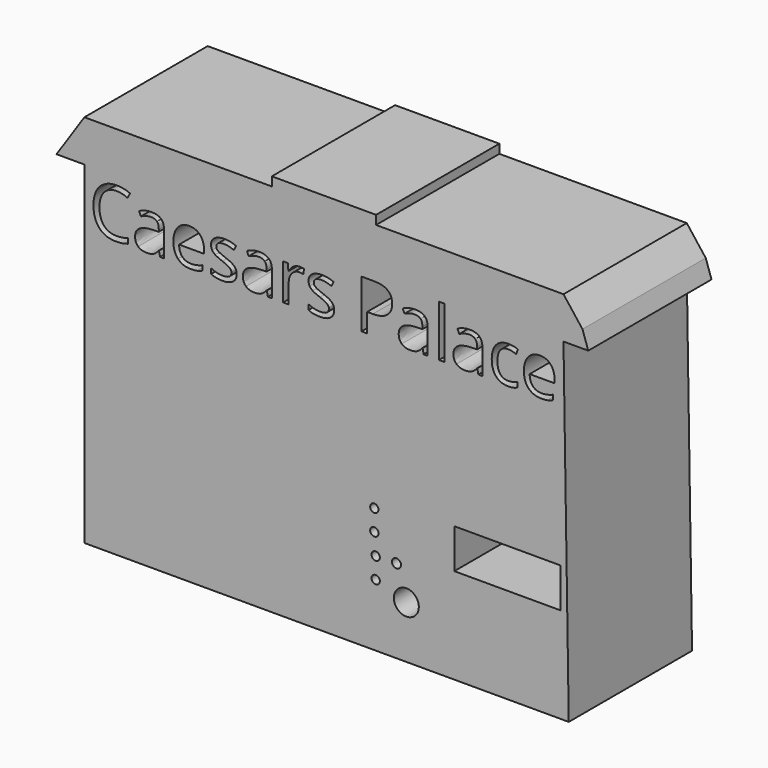
from build123d import *

# Parameters (mm, degrees)
F0_W     = 66.9038857644
F0_H     = 626.8855423356
F1_DEPTH = 1879.6
F2_R     = 54.9444288962
F2_R_2   = 50.8
F3_DEPTH = 4038.6
F4_W     = 1295.4
F4_H     = 482.6
F5_DEPTH = 2717.8
F6_R     = 152.4
F7_DEPTH = 3378.2


# Not quite as in the source:
# - a feature names something its author has since deleted; it is built from what else it names


with BuildPart() as f1:
    # F0 (on Front) → F1 (new body)
    with BuildSketch(Plane.XZ):
        Polygon((208.8753432035, -1016), (549.4310855865, -1016), (6393.364906311, -1016), (6695.2958106995, -1016), (6624.9423027039, -807.6888309717), (6393.364906311, -508), (4107.364906311, -508), (4107.364906311, -399.0220116377), (2835.4310855865, -399.0220116377), (2835.4310855865, -508), (549.4310855865, -508), align=None)
        Polygon((549.4310855865, -1016), (549.4310855865, -5080), (6457.6897621155, -5080), (6393.364906311, -1016), align=None)
        with BuildLine():
            add(Edge.make_bspline(
                [(1076.286761918, -1203.7427777217), (1009.3828761536, -1172.4178369881), (942.4789903892, -1172.4178369881)],
                knots=[0, 0, 0, 1, 1, 1], degree=2))
            add(Edge.make_bspline(
                [(942.4789903892, -1172.4178369881), (845.4103468814, -1172.4178369881), (789.2059264705, -1237.0658113828)],
                knots=[0, 0, 0, 1, 1, 1], degree=2))
            add(Edge.make_bspline(
                [(789.2059264705, -1237.0658113828), (733.0015060595, -1301.7137857775), (733.0015060595, -1414.1226265993)],
                knots=[0, 0, 0, 1, 1, 1], degree=2))
            add(Edge.make_bspline(
                [(733.0015060595, -1414.1226265993), (733.0015060595, -1529.6252887282), (787.207833543, -1592.7263524694)],
                knots=[0, 0, 0, 1, 1, 1], degree=2))
            add(Edge.make_bspline(
                [(787.207833543, -1592.7263524694), (841.4141610265, -1655.8274162105), (941.7055350625, -1655.8274162105)],
                knots=[0, 0, 0, 1, 1, 1], degree=2))
            add(Edge.make_bspline(
                [(941.7055350625, -1655.8274162105), (1003.3241427607, -1655.8274162105), (1082.3454953109, -1633.6550301769)],
                knots=[0, 0, 0, 1, 1, 1], degree=2))
            Line((1082.3454953109, -1633.6550301769), (1082.3454953109, -1693.5978180004))
            add(Edge.make_bspline(
                [(1082.3454953109, -1693.5978180004), (1021.1136152761, -1716.672568582), (931.2638881513, -1716.672568582)],
                knots=[0, 0, 0, 1, 1, 1], degree=2))
            add(Edge.make_bspline(
                [(931.2638881513, -1716.672568582), (801.1944840352, -1716.672568582), (730.4877762476, -1637.6512160318)],
                knots=[0, 0, 0, 1, 1, 1], degree=2))
            add(Edge.make_bspline(
                [(730.4877762476, -1637.6512160318), (659.78106846, -1558.6298634816), (659.78106846, -1413.2202620515)],
                knots=[0, 0, 0, 1, 1, 1], degree=2))
            add(Edge.make_bspline(
                [(659.78106846, -1413.2202620515), (659.78106846, -1322.2103519365), (693.8131028372, -1253.7595555186)],
                knots=[0, 0, 0, 1, 1, 1], degree=2))
            add(Edge.make_bspline(
                [(693.8131028372, -1253.7595555186), (727.8451372145, -1185.3087591007), (792.1063839458, -1148.247358027)],
                knots=[0, 0, 0, 1, 1, 1], degree=2))
            add(Edge.make_bspline(
                [(792.1063839458, -1148.247358027), (856.3676306771, -1111.1859569533), (943.3813549371, -1111.1859569533)],
                knots=[0, 0, 0, 1, 1, 1], degree=2))
            add(Edge.make_bspline(
                [(943.3813549371, -1111.1859569533), (1035.9381757056, -1111.1859569533), (1105.2913366713, -1144.9601728883)],
                knots=[0, 0, 0, 1, 1, 1], degree=2))
            Line((1105.2913366713, -1144.9601728883), (1076.286761918, -1203.7427777217))
        make_face(mode=Mode.SUBTRACT)
        with BuildLine():
            Line((1521.9259393505, -1708.5512876511), (1472.295889217, -1708.5512876511))
            Line((1472.295889217, -1708.5512876511), (1459.018239441, -1645.6435877416))
            Line((1459.018239441, -1645.6435877416), (1455.7955089129, -1645.6435877416))
            add(Edge.make_bspline(
                [(1455.7955089129, -1645.6435877416), (1422.7947483046, -1687.1523569442), (1389.9873515281, -1701.9124627631)],
                knots=[0, 0, 0, 1, 1, 1], degree=2))
            add(Edge.make_bspline(
                [(1389.9873515281, -1701.9124627631), (1357.1799547515, -1716.672568582), (1307.9366322814, -1716.672568582)],
                knots=[0, 0, 0, 1, 1, 1], degree=2))
            add(Edge.make_bspline(
                [(1307.9366322814, -1716.672568582), (1242.3218387283, -1716.672568582), (1205.0670738228, -1682.7694434259)],
                knots=[0, 0, 0, 1, 1, 1], degree=2))
            add(Edge.make_bspline(
                [(1205.0670738228, -1682.7694434259), (1167.8123089174, -1648.8663182697), (1167.8123089174, -1586.4742552448)],
                knots=[0, 0, 0, 1, 1, 1], degree=2))
            add(Edge.make_bspline(
                [(1167.8123089174, -1586.4742552448), (1167.8123089174, -1452.7953929371), (1381.6727067654, -1446.3499318808)],
                knots=[0, 0, 0, 1, 1, 1], degree=2))
            Line((1381.6727067654, -1446.3499318808), (1456.5689642396, -1443.9006566794))
            Line((1456.5689642396, -1443.9006566794), (1456.5689642396, -1416.4429925796))
            add(Edge.make_bspline(
                [(1456.5689642396, -1416.4429925796), (1456.5689642396, -1364.4925764658), (1434.2676689848, -1339.7420060097)],
                knots=[0, 0, 0, 1, 1, 1], degree=2))
            add(Edge.make_bspline(
                [(1434.2676689848, -1339.7420060097), (1411.96637373, -1314.9914355535), (1362.7230512599, -1314.9914355535)],
                knots=[0, 0, 0, 1, 1, 1], degree=2))
            add(Edge.make_bspline(
                [(1362.7230512599, -1314.9914355535), (1307.549904618, -1314.9914355535), (1237.93892521, -1348.7656514885)],
                knots=[0, 0, 0, 1, 1, 1], degree=2))
            Line((1237.93892521, -1348.7656514885), (1217.3134498298, -1297.5886907015))
            add(Edge.make_bspline(
                [(1217.3134498298, -1297.5886907015), (1249.9274827747, -1279.9281274072), (1288.7936129442, -1269.8732081594)],
                knots=[0, 0, 0, 1, 1, 1], degree=2))
            add(Edge.make_bspline(
                [(1288.7936129442, -1269.8732081594), (1327.6597431137, -1259.8182889115), (1366.8481463359, -1259.8182889115)],
                knots=[0, 0, 0, 1, 1, 1], degree=2))
            add(Edge.make_bspline(
                [(1366.8481463359, -1259.8182889115), (1445.740589665, -1259.8182889115), (1483.8332645078, -1294.8171424472)],
                knots=[0, 0, 0, 1, 1, 1], degree=2))
            add(Edge.make_bspline(
                [(1483.8332645078, -1294.8171424472), (1521.9259393505, -1329.815995983), (1521.9259393505, -1407.1615286585)],
                knots=[0, 0, 0, 1, 1, 1], degree=2))
            Line((1521.9259393505, -1407.1615286585), (1521.9259393505, -1708.5512876511))
        make_face(mode=Mode.SUBTRACT)
        with BuildLine():
            add(Edge.make_bspline(
                [(1922.4468893889, -1709.9692890834), (1890.864130213, -1716.672568582), (1846.1326304823, -1716.672568582)],
                knots=[0, 0, 0, 1, 1, 1], degree=2))
            add(Edge.make_bspline(
                [(1846.1326304823, -1716.672568582), (1748.2905316477, -1716.672568582), (1691.6349289628, -1656.9875992007)],
                knots=[0, 0, 0, 1, 1, 1], degree=2))
            add(Edge.make_bspline(
                [(1691.6349289628, -1656.9875992007), (1634.979326278, -1597.3026298193), (1634.979326278, -1491.4681592749)],
                knots=[0, 0, 0, 1, 1, 1], degree=2))
            add(Edge.make_bspline(
                [(1634.979326278, -1491.4681592749), (1634.979326278, -1384.6024149615), (1687.5742884974, -1321.7591696626)],
                knots=[0, 0, 0, 1, 1, 1], degree=2))
            add(Edge.make_bspline(
                [(1687.5742884974, -1321.7591696626), (1740.1692507168, -1258.9159243637), (1828.8587948514, -1258.9159243637)],
                knots=[0, 0, 0, 1, 1, 1], degree=2))
            add(Edge.make_bspline(
                [(1828.8587948514, -1258.9159243637), (1911.7474240354, -1258.9159243637), (1960.0883819577, -1313.5089795105)],
                knots=[0, 0, 0, 1, 1, 1], degree=2))
            add(Edge.make_bspline(
                [(1960.0883819577, -1313.5089795105), (2008.4293398799, -1368.1020346574), (2008.4293398799, -1457.5650341188)],
                knots=[0, 0, 0, 1, 1, 1], degree=2))
            Line((2008.4293398799, -1457.5650341188), (2008.4293398799, -1499.8472586481))
            Line((2008.4293398799, -1499.8472586481), (1704.3324872437, -1499.8472586481))
            add(Edge.make_bspline(
                [(1704.3324872437, -1499.8472586481), (1706.3950347818, -1577.5795189871), (1743.6497996872, -1617.8636505889)],
                knots=[0, 0, 0, 1, 1, 1], degree=2))
            add(Edge.make_bspline(
                [(1743.6497996872, -1617.8636505889), (1780.9045645926, -1658.1477821908), (1848.5819056837, -1658.1477821908)],
                knots=[0, 0, 0, 1, 1, 1], degree=2))
            add(Edge.make_bspline(
                [(1848.5819056837, -1658.1477821908), (1919.8687049664, -1658.1477821908), (1989.4796843744, -1628.3697521107)],
                knots=[0, 0, 0, 1, 1, 1], degree=2))
            Line((1989.4796843744, -1628.3697521107), (1989.4796843744, -1688.054721492))
            add(Edge.make_bspline(
                [(1989.4796843744, -1688.054721492), (1954.0296485648, -1703.2660095849), (1922.4468893889, -1709.9692890834)],
                knots=[0, 0, 0, 1, 1, 1], degree=2))
        make_face(mode=Mode.SUBTRACT)
        with BuildLine():
            add(Edge.make_bspline(
                [(2379.6878967227, -1515.1874559621), (2407.2744700437, -1544.1920307154), (2407.2744700437, -1588.1500751194)],
                knots=[0, 0, 0, 1, 1, 1], degree=2))
            add(Edge.make_bspline(
                [(2407.2744700437, -1588.1500751194), (2407.2744700437, -1649.7686828176), (2361.3827873228, -1683.2206256998)],
                knots=[0, 0, 0, 1, 1, 1], degree=2))
            add(Edge.make_bspline(
                [(2361.3827873228, -1683.2206256998), (2315.491104602, -1716.672568582), (2232.4735661969, -1716.672568582)],
                knots=[0, 0, 0, 1, 1, 1], degree=2))
            add(Edge.make_bspline(
                [(2232.4735661969, -1716.672568582), (2144.6863866101, -1716.672568582), (2095.5719733611, -1688.8281768188)],
                knots=[0, 0, 0, 1, 1, 1], degree=2))
            Line((2095.5719733611, -1688.8281768188), (2095.5719733611, -1626.8228414572))
            add(Edge.make_bspline(
                [(2095.5719733611, -1626.8228414572), (2127.4125509792, -1642.9364940979), (2163.8294059473, -1652.1535034084)],
                knots=[0, 0, 0, 1, 1, 1], degree=2))
            add(Edge.make_bspline(
                [(2163.8294059473, -1652.1535034084), (2200.2462609154, -1661.370512719), (2234.1493860715, -1661.370512719)],
                knots=[0, 0, 0, 1, 1, 1], degree=2))
            add(Edge.make_bspline(
                [(2234.1493860715, -1661.370512719), (2286.4865298486, -1661.370512719), (2314.6531946647, -1644.6767685831)],
                knots=[0, 0, 0, 1, 1, 1], degree=2))
            add(Edge.make_bspline(
                [(2314.6531946647, -1644.6767685831), (2342.8198594807, -1627.9830244473), (2342.8198594807, -1593.6931716278)],
                knots=[0, 0, 0, 1, 1, 1], degree=2))
            add(Edge.make_bspline(
                [(2342.8198594807, -1593.6931716278), (2342.8198594807, -1567.9113274026), (2320.5185642259, -1549.6062180027)],
                knots=[0, 0, 0, 1, 1, 1], degree=2))
            add(Edge.make_bspline(
                [(2320.5185642259, -1549.6062180027), (2298.2172689711, -1531.3011086028), (2233.2470215236, -1506.2927197044)],
                knots=[0, 0, 0, 1, 1, 1], degree=2))
            add(Edge.make_bspline(
                [(2233.2470215236, -1506.2927197044), (2171.6284138254, -1483.346878344), (2145.6532057685, -1466.2019519342)],
                knots=[0, 0, 0, 1, 1, 1], degree=2))
            add(Edge.make_bspline(
                [(2145.6532057685, -1466.2019519342), (2119.6779977116, -1449.0570255245), (2106.9804394307, -1427.3358217648)],
                knots=[0, 0, 0, 1, 1, 1], degree=2))
            add(Edge.make_bspline(
                [(2106.9804394307, -1427.3358217648), (2094.2828811498, -1405.614618005), (2094.2828811498, -1375.4498602615)],
                knots=[0, 0, 0, 1, 1, 1], degree=2))
            add(Edge.make_bspline(
                [(2094.2828811498, -1375.4498602615), (2094.2828811498, -1321.4368966098), (2138.2409255538, -1290.1764104867)],
                knots=[0, 0, 0, 1, 1, 1], degree=2))
            add(Edge.make_bspline(
                [(2138.2409255538, -1290.1764104867), (2182.1989699577, -1258.9159243637), (2258.6421380854, -1258.9159243637)],
                knots=[0, 0, 0, 1, 1, 1], degree=2))
            add(Edge.make_bspline(
                [(2258.6421380854, -1258.9159243637), (2329.9289373681, -1258.9159243637), (2398.1219153437, -1287.920499117)],
                knots=[0, 0, 0, 1, 1, 1], degree=2))
            Line((2398.1219153437, -1287.920499117), (2374.2737094354, -1342.3201904322))
            add(Edge.make_bspline(
                [(2374.2737094354, -1342.3201904322), (2307.8854605556, -1314.9914355535), (2253.8724969038, -1314.9914355535)],
                knots=[0, 0, 0, 1, 1, 1], degree=2))
            add(Edge.make_bspline(
                [(2253.8724969038, -1314.9914355535), (2206.3049943083, -1314.9914355535), (2182.1345153472, -1329.8804505935)],
                knots=[0, 0, 0, 1, 1, 1], degree=2))
            add(Edge.make_bspline(
                [(2182.1345153472, -1329.8804505935), (2157.964036386, -1344.7694656336), (2157.964036386, -1370.9380375221)],
                knots=[0, 0, 0, 1, 1, 1], degree=2))
            add(Edge.make_bspline(
                [(2157.964036386, -1370.9380375221), (2157.964036386, -1388.7275100375), (2167.0521364754, -1401.1672498762)],
                knots=[0, 0, 0, 1, 1, 1], degree=2))
            add(Edge.make_bspline(
                [(2167.0521364754, -1401.1672498762), (2176.1402365648, -1413.6069897148), (2196.2500750605, -1424.8865465634)],
                knots=[0, 0, 0, 1, 1, 1], degree=2))
            add(Edge.make_bspline(
                [(2196.2500750605, -1424.8865465634), (2216.3599135561, -1436.1661034119), (2273.595607736, -1457.5650341188)],
                knots=[0, 0, 0, 1, 1, 1], degree=2))
            add(Edge.make_bspline(
                [(2273.595607736, -1457.5650341188), (2352.1013234018, -1486.1828812088), (2379.6878967227, -1515.1874559621)],
                knots=[0, 0, 0, 1, 1, 1], degree=2))
        make_face(mode=Mode.SUBTRACT)
        with BuildLine():
            Line((2837.1867224988, -1708.5512876511), (2787.5566723653, -1708.5512876511))
            Line((2787.5566723653, -1708.5512876511), (2774.2790225893, -1645.6435877416))
            Line((2774.2790225893, -1645.6435877416), (2771.0562920612, -1645.6435877416))
            add(Edge.make_bspline(
                [(2771.0562920612, -1645.6435877416), (2738.0555314529, -1687.1523569442), (2705.2481346764, -1701.9124627631)],
                knots=[0, 0, 0, 1, 1, 1], degree=2))
            add(Edge.make_bspline(
                [(2705.2481346764, -1701.9124627631), (2672.4407378998, -1716.672568582), (2623.1974154297, -1716.672568582)],
                knots=[0, 0, 0, 1, 1, 1], degree=2))
            add(Edge.make_bspline(
                [(2623.1974154297, -1716.672568582), (2557.5826218766, -1716.672568582), (2520.3278569712, -1682.7694434259)],
                knots=[0, 0, 0, 1, 1, 1], degree=2))
            add(Edge.make_bspline(
                [(2520.3278569712, -1682.7694434259), (2483.0730920658, -1648.8663182697), (2483.0730920658, -1586.4742552448)],
                knots=[0, 0, 0, 1, 1, 1], degree=2))
            add(Edge.make_bspline(
                [(2483.0730920658, -1586.4742552448), (2483.0730920658, -1452.7953929371), (2696.9334899137, -1446.3499318808)],
                knots=[0, 0, 0, 1, 1, 1], degree=2))
            Line((2696.9334899137, -1446.3499318808), (2771.8297473879, -1443.9006566794))
            Line((2771.8297473879, -1443.9006566794), (2771.8297473879, -1416.4429925796))
            add(Edge.make_bspline(
                [(2771.8297473879, -1416.4429925796), (2771.8297473879, -1364.4925764658), (2749.5284521331, -1339.7420060097)],
                knots=[0, 0, 0, 1, 1, 1], degree=2))
            add(Edge.make_bspline(
                [(2749.5284521331, -1339.7420060097), (2727.2271568783, -1314.9914355535), (2677.9838344082, -1314.9914355535)],
                knots=[0, 0, 0, 1, 1, 1], degree=2))
            add(Edge.make_bspline(
                [(2677.9838344082, -1314.9914355535), (2622.8106877663, -1314.9914355535), (2553.1997083583, -1348.7656514885)],
                knots=[0, 0, 0, 1, 1, 1], degree=2))
            Line((2553.1997083583, -1348.7656514885), (2532.5742329781, -1297.5886907015))
            add(Edge.make_bspline(
                [(2532.5742329781, -1297.5886907015), (2565.188265923, -1279.9281274072), (2604.0543960925, -1269.8732081594)],
                knots=[0, 0, 0, 1, 1, 1], degree=2))
            add(Edge.make_bspline(
                [(2604.0543960925, -1269.8732081594), (2642.920526262, -1259.8182889115), (2682.1089294843, -1259.8182889115)],
                knots=[0, 0, 0, 1, 1, 1], degree=2))
            add(Edge.make_bspline(
                [(2682.1089294843, -1259.8182889115), (2761.0013728134, -1259.8182889115), (2799.0940476561, -1294.8171424472)],
                knots=[0, 0, 0, 1, 1, 1], degree=2))
            add(Edge.make_bspline(
                [(2799.0940476561, -1294.8171424472), (2837.1867224988, -1329.815995983), (2837.1867224988, -1407.1615286585)],
                knots=[0, 0, 0, 1, 1, 1], degree=2))
            Line((2837.1867224988, -1407.1615286585), (2837.1867224988, -1708.5512876511))
        make_face(mode=Mode.SUBTRACT)
        with BuildLine():
            add(Edge.make_bspline(
                [(3100.1615335958, -1282.312947998), (3134.8381140787, -1258.9159243637), (3176.3468832812, -1258.9159243637)],
                knots=[0, 0, 0, 1, 1, 1], degree=2))
            add(Edge.make_bspline(
                [(3176.3468832812, -1258.9159243637), (3205.738185698, -1258.9159243637), (3229.0707547218, -1263.8144747665)],
                knots=[0, 0, 0, 1, 1, 1], degree=2))
            Line((3229.0707547218, -1263.8144747665), (3219.7892908007, -1325.819810128))
            add(Edge.make_bspline(
                [(3219.7892908007, -1325.819810128), (3192.460535922, -1319.7610767351), (3171.4483328785, -1319.7610767351)],
                knots=[0, 0, 0, 1, 1, 1], degree=2))
            add(Edge.make_bspline(
                [(3171.4483328785, -1319.7610767351), (3117.82209689, -1319.7610767351), (3079.7938766579, -1363.2679388651)],
                knots=[0, 0, 0, 1, 1, 1], degree=2))
            add(Edge.make_bspline(
                [(3079.7938766579, -1363.2679388651), (3041.7656564257, -1406.7748009952), (3041.7656564257, -1471.6161392215)],
                knots=[0, 0, 0, 1, 1, 1], degree=2))
            Line((3041.7656564257, -1471.6161392215), (3041.7656564257, -1708.5512876511))
            Line((3041.7656564257, -1708.5512876511), (2974.8617706613, -1708.5512876511))
            Line((2974.8617706613, -1708.5512876511), (2974.8617706613, -1267.0372052946))
            Line((2974.8617706613, -1267.0372052946), (3030.0349173033, -1267.0372052946))
            Line((3030.0349173033, -1267.0372052946), (3037.7694705708, -1348.7656514885))
            Line((3037.7694705708, -1348.7656514885), (3040.992201099, -1348.7656514885))
            add(Edge.make_bspline(
                [(3040.992201099, -1348.7656514885), (3065.4849531129, -1305.7099716324), (3100.1615335958, -1282.312947998)],
                knots=[0, 0, 0, 1, 1, 1], degree=2))
        make_face(mode=Mode.SUBTRACT)
        with BuildLine():
            add(Edge.make_bspline(
                [(3568.8754616098, -1515.1874559621), (3596.4620349308, -1544.1920307154), (3596.4620349308, -1588.1500751194)],
                knots=[0, 0, 0, 1, 1, 1], degree=2))
            add(Edge.make_bspline(
                [(3596.4620349308, -1588.1500751194), (3596.4620349308, -1649.7686828176), (3550.5703522099, -1683.2206256998)],
                knots=[0, 0, 0, 1, 1, 1], degree=2))
            add(Edge.make_bspline(
                [(3550.5703522099, -1683.2206256998), (3504.6786694891, -1716.672568582), (3421.661131084, -1716.672568582)],
                knots=[0, 0, 0, 1, 1, 1], degree=2))
            add(Edge.make_bspline(
                [(3421.661131084, -1716.672568582), (3333.8739514972, -1716.672568582), (3284.7595382482, -1688.8281768188)],
                knots=[0, 0, 0, 1, 1, 1], degree=2))
            Line((3284.7595382482, -1688.8281768188), (3284.7595382482, -1626.8228414572))
            add(Edge.make_bspline(
                [(3284.7595382482, -1626.8228414572), (3316.6001158663, -1642.9364940979), (3353.0169708344, -1652.1535034084)],
                knots=[0, 0, 0, 1, 1, 1], degree=2))
            add(Edge.make_bspline(
                [(3353.0169708344, -1652.1535034084), (3389.4338258025, -1661.370512719), (3423.3369509586, -1661.370512719)],
                knots=[0, 0, 0, 1, 1, 1], degree=2))
            add(Edge.make_bspline(
                [(3423.3369509586, -1661.370512719), (3475.6740947358, -1661.370512719), (3503.8407595518, -1644.6767685831)],
                knots=[0, 0, 0, 1, 1, 1], degree=2))
            add(Edge.make_bspline(
                [(3503.8407595518, -1644.6767685831), (3532.0074243678, -1627.9830244473), (3532.0074243678, -1593.6931716278)],
                knots=[0, 0, 0, 1, 1, 1], degree=2))
            add(Edge.make_bspline(
                [(3532.0074243678, -1593.6931716278), (3532.0074243678, -1567.9113274026), (3509.706129113, -1549.6062180027)],
                knots=[0, 0, 0, 1, 1, 1], degree=2))
            add(Edge.make_bspline(
                [(3509.706129113, -1549.6062180027), (3487.4048338582, -1531.3011086028), (3422.4345864107, -1506.2927197044)],
                knots=[0, 0, 0, 1, 1, 1], degree=2))
            add(Edge.make_bspline(
                [(3422.4345864107, -1506.2927197044), (3360.8159787125, -1483.346878344), (3334.8407706556, -1466.2019519342)],
                knots=[0, 0, 0, 1, 1, 1], degree=2))
            add(Edge.make_bspline(
                [(3334.8407706556, -1466.2019519342), (3308.8655625987, -1449.0570255245), (3296.1680043178, -1427.3358217648)],
                knots=[0, 0, 0, 1, 1, 1], degree=2))
            add(Edge.make_bspline(
                [(3296.1680043178, -1427.3358217648), (3283.4704460369, -1405.614618005), (3283.4704460369, -1375.4498602615)],
                knots=[0, 0, 0, 1, 1, 1], degree=2))
            add(Edge.make_bspline(
                [(3283.4704460369, -1375.4498602615), (3283.4704460369, -1321.4368966098), (3327.4284904409, -1290.1764104867)],
                knots=[0, 0, 0, 1, 1, 1], degree=2))
            add(Edge.make_bspline(
                [(3327.4284904409, -1290.1764104867), (3371.3865348448, -1258.9159243637), (3447.8297029725, -1258.9159243637)],
                knots=[0, 0, 0, 1, 1, 1], degree=2))
            add(Edge.make_bspline(
                [(3447.8297029725, -1258.9159243637), (3519.1165022552, -1258.9159243637), (3587.3094802308, -1287.920499117)],
                knots=[0, 0, 0, 1, 1, 1], degree=2))
            Line((3587.3094802308, -1287.920499117), (3563.4612743225, -1342.3201904322))
            add(Edge.make_bspline(
                [(3563.4612743225, -1342.3201904322), (3497.0730254427, -1314.9914355535), (3443.0600617909, -1314.9914355535)],
                knots=[0, 0, 0, 1, 1, 1], degree=2))
            add(Edge.make_bspline(
                [(3443.0600617909, -1314.9914355535), (3395.4925591954, -1314.9914355535), (3371.3220802343, -1329.8804505935)],
                knots=[0, 0, 0, 1, 1, 1], degree=2))
            add(Edge.make_bspline(
                [(3371.3220802343, -1329.8804505935), (3347.1516012732, -1344.7694656336), (3347.1516012732, -1370.9380375221)],
                knots=[0, 0, 0, 1, 1, 1], degree=2))
            add(Edge.make_bspline(
                [(3347.1516012732, -1370.9380375221), (3347.1516012732, -1388.7275100375), (3356.2397013625, -1401.1672498762)],
                knots=[0, 0, 0, 1, 1, 1], degree=2))
            add(Edge.make_bspline(
                [(3356.2397013625, -1401.1672498762), (3365.3278014519, -1413.6069897148), (3385.4376399476, -1424.8865465634)],
                knots=[0, 0, 0, 1, 1, 1], degree=2))
            add(Edge.make_bspline(
                [(3385.4376399476, -1424.8865465634), (3405.5474784432, -1436.1661034119), (3462.7831726232, -1457.5650341188)],
                knots=[0, 0, 0, 1, 1, 1], degree=2))
            add(Edge.make_bspline(
                [(3462.7831726232, -1457.5650341188), (3541.2888882889, -1486.1828812088), (3568.8754616098, -1515.1874559621)],
                knots=[0, 0, 0, 1, 1, 1], degree=2))
        make_face(mode=Mode.SUBTRACT)
        with BuildLine():
            add(Edge.make_bspline(
                [(4082.4497985757, -1119.5650563265), (4303.1423851434, -1119.5650563265), (4303.1423851434, -1291.1432296452)],
                knots=[0, 0, 0, 1, 1, 1], degree=2))
            add(Edge.make_bspline(
                [(4303.1423851434, -1291.1432296452), (4303.1423851434, -1380.6062291066), (4242.1038689402, -1428.7538231971)],
                knots=[0, 0, 0, 1, 1, 1], degree=2))
            add(Edge.make_bspline(
                [(4242.1038689402, -1428.7538231971), (4181.0653527371, -1476.9014172877), (4067.4963289251, -1476.9014172877)],
                knots=[0, 0, 0, 1, 1, 1], degree=2))
            Line((4067.4963289251, -1476.9014172877), (3998.1431679593, -1476.9014172877))
            Line((3998.1431679593, -1476.9014172877), (3998.1431679593, -1708.5512876511))
            Line((3998.1431679593, -1708.5512876511), (3929.6923715414, -1708.5512876511))
            Line((3929.6923715414, -1708.5512876511), (3929.6923715414, -1119.5650563265))
            Line((3929.6923715414, -1119.5650563265), (4082.4497985757, -1119.5650563265))
        make_face(mode=Mode.SUBTRACT)
        with BuildLine():
            Line((4737.4375511168, -1708.5512876511), (4687.8075009833, -1708.5512876511))
            Line((4687.8075009833, -1708.5512876511), (4674.5298512073, -1645.6435877416))
            Line((4674.5298512073, -1645.6435877416), (4671.3071206792, -1645.6435877416))
            add(Edge.make_bspline(
                [(4671.3071206792, -1645.6435877416), (4638.3063600709, -1687.1523569442), (4605.4989632943, -1701.9124627631)],
                knots=[0, 0, 0, 1, 1, 1], degree=2))
            add(Edge.make_bspline(
                [(4605.4989632943, -1701.9124627631), (4572.6915665178, -1716.672568582), (4523.4482440477, -1716.672568582)],
                knots=[0, 0, 0, 1, 1, 1], degree=2))
            add(Edge.make_bspline(
                [(4523.4482440477, -1716.672568582), (4457.8334504945, -1716.672568582), (4420.5786855891, -1682.7694434259)],
                knots=[0, 0, 0, 1, 1, 1], degree=2))
            add(Edge.make_bspline(
                [(4420.5786855891, -1682.7694434259), (4383.3239206837, -1648.8663182697), (4383.3239206837, -1586.4742552448)],
                knots=[0, 0, 0, 1, 1, 1], degree=2))
            add(Edge.make_bspline(
                [(4383.3239206837, -1586.4742552448), (4383.3239206837, -1452.7953929371), (4597.1843185317, -1446.3499318808)],
                knots=[0, 0, 0, 1, 1, 1], degree=2))
            Line((4597.1843185317, -1446.3499318808), (4672.0805760059, -1443.9006566794))
            Line((4672.0805760059, -1443.9006566794), (4672.0805760059, -1416.4429925796))
            add(Edge.make_bspline(
                [(4672.0805760059, -1416.4429925796), (4672.0805760059, -1364.4925764658), (4649.7792807511, -1339.7420060097)],
                knots=[0, 0, 0, 1, 1, 1], degree=2))
            add(Edge.make_bspline(
                [(4649.7792807511, -1339.7420060097), (4627.4779854963, -1314.9914355535), (4578.2346630262, -1314.9914355535)],
                knots=[0, 0, 0, 1, 1, 1], degree=2))
            add(Edge.make_bspline(
                [(4578.2346630262, -1314.9914355535), (4523.0615163843, -1314.9914355535), (4453.4505369763, -1348.7656514885)],
                knots=[0, 0, 0, 1, 1, 1], degree=2))
            Line((4453.4505369763, -1348.7656514885), (4432.8250615961, -1297.5886907015))
            add(Edge.make_bspline(
                [(4432.8250615961, -1297.5886907015), (4465.439094541, -1279.9281274072), (4504.3052247105, -1269.8732081594)],
                knots=[0, 0, 0, 1, 1, 1], degree=2))
            add(Edge.make_bspline(
                [(4504.3052247105, -1269.8732081594), (4543.1713548799, -1259.8182889115), (4582.3597581022, -1259.8182889115)],
                knots=[0, 0, 0, 1, 1, 1], degree=2))
            add(Edge.make_bspline(
                [(4582.3597581022, -1259.8182889115), (4661.2522014313, -1259.8182889115), (4699.3448762741, -1294.8171424472)],
                knots=[0, 0, 0, 1, 1, 1], degree=2))
            add(Edge.make_bspline(
                [(4699.3448762741, -1294.8171424472), (4737.4375511168, -1329.815995983), (4737.4375511168, -1407.1615286585)],
                knots=[0, 0, 0, 1, 1, 1], degree=2))
            Line((4737.4375511168, -1407.1615286585), (4737.4375511168, -1708.5512876511))
        make_face(mode=Mode.SUBTRACT)
        with Locations((4908.5645421615, -1395.1085164833)):
            Rectangle(F0_W, F0_H, mode=Mode.SUBTRACT)
        with BuildLine():
            Line((5404.9294981071, -1708.5512876511), (5355.2994479736, -1708.5512876511))
            Line((5355.2994479736, -1708.5512876511), (5342.0217981976, -1645.6435877416))
            Line((5342.0217981976, -1645.6435877416), (5338.7990676694, -1645.6435877416))
            add(Edge.make_bspline(
                [(5338.7990676694, -1645.6435877416), (5305.7983070612, -1687.1523569442), (5272.9909102846, -1701.9124627631)],
                knots=[0, 0, 0, 1, 1, 1], degree=2))
            add(Edge.make_bspline(
                [(5272.9909102846, -1701.9124627631), (5240.1835135081, -1716.672568582), (5190.940191038, -1716.672568582)],
                knots=[0, 0, 0, 1, 1, 1], degree=2))
            add(Edge.make_bspline(
                [(5190.940191038, -1716.672568582), (5125.3253974848, -1716.672568582), (5088.0706325794, -1682.7694434259)],
                knots=[0, 0, 0, 1, 1, 1], degree=2))
            add(Edge.make_bspline(
                [(5088.0706325794, -1682.7694434259), (5050.815867674, -1648.8663182697), (5050.815867674, -1586.4742552448)],
                knots=[0, 0, 0, 1, 1, 1], degree=2))
            add(Edge.make_bspline(
                [(5050.815867674, -1586.4742552448), (5050.815867674, -1452.7953929371), (5264.676265522, -1446.3499318808)],
                knots=[0, 0, 0, 1, 1, 1], degree=2))
            Line((5264.676265522, -1446.3499318808), (5339.5725229962, -1443.9006566794))
            Line((5339.5725229962, -1443.9006566794), (5339.5725229962, -1416.4429925796))
            add(Edge.make_bspline(
                [(5339.5725229962, -1416.4429925796), (5339.5725229962, -1364.4925764658), (5317.2712277414, -1339.7420060097)],
                knots=[0, 0, 0, 1, 1, 1], degree=2))
            add(Edge.make_bspline(
                [(5317.2712277414, -1339.7420060097), (5294.9699324866, -1314.9914355535), (5245.7266100165, -1314.9914355535)],
                knots=[0, 0, 0, 1, 1, 1], degree=2))
            add(Edge.make_bspline(
                [(5245.7266100165, -1314.9914355535), (5190.5534633746, -1314.9914355535), (5120.9424839666, -1348.7656514885)],
                knots=[0, 0, 0, 1, 1, 1], degree=2))
            Line((5120.9424839666, -1348.7656514885), (5100.3170085864, -1297.5886907015))
            add(Edge.make_bspline(
                [(5100.3170085864, -1297.5886907015), (5132.9310415313, -1279.9281274072), (5171.7971717007, -1269.8732081594)],
                knots=[0, 0, 0, 1, 1, 1], degree=2))
            add(Edge.make_bspline(
                [(5171.7971717007, -1269.8732081594), (5210.6633018702, -1259.8182889115), (5249.8517050925, -1259.8182889115)],
                knots=[0, 0, 0, 1, 1, 1], degree=2))
            add(Edge.make_bspline(
                [(5249.8517050925, -1259.8182889115), (5328.7441484216, -1259.8182889115), (5366.8368232643, -1294.8171424472)],
                knots=[0, 0, 0, 1, 1, 1], degree=2))
            add(Edge.make_bspline(
                [(5366.8368232643, -1294.8171424472), (5404.9294981071, -1329.815995983), (5404.9294981071, -1407.1615286585)],
                knots=[0, 0, 0, 1, 1, 1], degree=2))
            Line((5404.9294981071, -1407.1615286585), (5404.9294981071, -1708.5512876511))
        make_face(mode=Mode.SUBTRACT)
        with BuildLine():
            add(Edge.make_bspline(
                [(5830.587746265, -1693.5978180004), (5786.3718834188, -1716.672568582), (5719.0812699911, -1716.672568582)],
                knots=[0, 0, 0, 1, 1, 1], degree=2))
            add(Edge.make_bspline(
                [(5719.0812699911, -1716.672568582), (5623.1728094733, -1716.672568582), (5570.5778472539, -1657.6321453063)],
                knots=[0, 0, 0, 1, 1, 1], degree=2))
            add(Edge.make_bspline(
                [(5570.5778472539, -1657.6321453063), (5517.9828850346, -1598.5917220306), (5517.9828850346, -1490.565794727)],
                knots=[0, 0, 0, 1, 1, 1], degree=2))
            add(Edge.make_bspline(
                [(5517.9828850346, -1490.565794727), (5517.9828850346, -1379.8327737798), (5571.4157571913, -1319.3743490717)],
                knots=[0, 0, 0, 1, 1, 1], degree=2))
            add(Edge.make_bspline(
                [(5571.4157571913, -1319.3743490717), (5624.848629348, -1258.9159243637), (5723.4641835094, -1258.9159243637)],
                knots=[0, 0, 0, 1, 1, 1], degree=2))
            add(Edge.make_bspline(
                [(5723.4641835094, -1258.9159243637), (5755.3047611275, -1258.9159243637), (5787.1453387456, -1265.8125676939)],
                knots=[0, 0, 0, 1, 1, 1], degree=2))
            add(Edge.make_bspline(
                [(5787.1453387456, -1265.8125676939), (5818.9859163637, -1272.7092110241), (5837.0332073213, -1281.9906749452)],
                knots=[0, 0, 0, 1, 1, 1], degree=2))
            Line((5837.0332073213, -1281.9906749452), (5816.5366411623, -1338.7107322406))
            add(Edge.make_bspline(
                [(5816.5366411623, -1338.7107322406), (5794.3642551286, -1329.815995983), (5768.1956832401, -1324.0150810323)],
                knots=[0, 0, 0, 1, 1, 1], degree=2))
            add(Edge.make_bspline(
                [(5768.1956832401, -1324.0150810323), (5742.0271113515, -1318.2141660816), (5721.9172728558, -1318.2141660816)],
                knots=[0, 0, 0, 1, 1, 1], degree=2))
            add(Edge.make_bspline(
                [(5721.9172728558, -1318.2141660816), (5587.3360460003, -1318.2141660816), (5587.3360460003, -1489.7923394003)],
                knots=[0, 0, 0, 1, 1, 1], degree=2))
            add(Edge.make_bspline(
                [(5587.3360460003, -1489.7923394003), (5587.3360460003, -1571.1340579308), (5620.1434427769, -1614.6409200608)],
                knots=[0, 0, 0, 1, 1, 1], degree=2))
            add(Edge.make_bspline(
                [(5620.1434427769, -1614.6409200608), (5652.9508395534, -1658.1477821908), (5717.4054501164, -1658.1477821908)],
                knots=[0, 0, 0, 1, 1, 1], degree=2))
            add(Edge.make_bspline(
                [(5717.4054501164, -1658.1477821908), (5772.5785967583, -1658.1477821908), (5830.587746265, -1634.4284855036)],
                knots=[0, 0, 0, 1, 1, 1], degree=2))
            Line((5830.587746265, -1634.4284855036), (5830.587746265, -1693.5978180004))
        make_face(mode=Mode.SUBTRACT)
        with BuildLine():
            add(Edge.make_bspline(
                [(6198.2368449163, -1709.9692890834), (6166.6540857405, -1716.672568582), (6121.9225860097, -1716.672568582)],
                knots=[0, 0, 0, 1, 1, 1], degree=2))
            add(Edge.make_bspline(
                [(6121.9225860097, -1716.672568582), (6024.0804871751, -1716.672568582), (5967.4248844903, -1656.9875992007)],
                knots=[0, 0, 0, 1, 1, 1], degree=2))
            add(Edge.make_bspline(
                [(5967.4248844903, -1656.9875992007), (5910.7692818054, -1597.3026298193), (5910.7692818054, -1491.4681592749)],
                knots=[0, 0, 0, 1, 1, 1], degree=2))
            add(Edge.make_bspline(
                [(5910.7692818054, -1491.4681592749), (5910.7692818054, -1384.6024149615), (5963.3642440248, -1321.7591696626)],
                knots=[0, 0, 0, 1, 1, 1], degree=2))
            add(Edge.make_bspline(
                [(5963.3642440248, -1321.7591696626), (6015.9592062442, -1258.9159243637), (6104.6487503789, -1258.9159243637)],
                knots=[0, 0, 0, 1, 1, 1], degree=2))
            add(Edge.make_bspline(
                [(6104.6487503789, -1258.9159243637), (6187.5373795629, -1258.9159243637), (6235.8783374851, -1313.5089795105)],
                knots=[0, 0, 0, 1, 1, 1], degree=2))
            add(Edge.make_bspline(
                [(6235.8783374851, -1313.5089795105), (6284.2192954073, -1368.1020346574), (6284.2192954073, -1457.5650341188)],
                knots=[0, 0, 0, 1, 1, 1], degree=2))
            Line((6284.2192954073, -1457.5650341188), (6284.2192954073, -1499.8472586481))
            Line((6284.2192954073, -1499.8472586481), (5980.1224427712, -1499.8472586481))
            add(Edge.make_bspline(
                [(5980.1224427712, -1499.8472586481), (5982.1849903092, -1577.5795189871), (6019.4397552146, -1617.8636505889)],
                knots=[0, 0, 0, 1, 1, 1], degree=2))
            add(Edge.make_bspline(
                [(6019.4397552146, -1617.8636505889), (6056.69452012, -1658.1477821908), (6124.3718612111, -1658.1477821908)],
                knots=[0, 0, 0, 1, 1, 1], degree=2))
            add(Edge.make_bspline(
                [(6124.3718612111, -1658.1477821908), (6195.6586604938, -1658.1477821908), (6265.2696399018, -1628.3697521107)],
                knots=[0, 0, 0, 1, 1, 1], degree=2))
            Line((6265.2696399018, -1628.3697521107), (6265.2696399018, -1688.054721492))
            add(Edge.make_bspline(
                [(6265.2696399018, -1688.054721492), (6229.8196040922, -1703.2660095849), (6198.2368449163, -1709.9692890834)],
                knots=[0, 0, 0, 1, 1, 1], degree=2))
        make_face(mode=Mode.SUBTRACT)
    extrude(amount=F1_DEPTH)

    # F2 (on face) → F3 (cut)
    with BuildSketch(Plane.XZ.offset(1879.6)):
        with Locations((4356.5925237601, -4060.8731475131)):
            Circle(F2_R)
        with Locations((4086.0152244568, -3810.3141784668)):
            Circle(F2_R_2)
        with Locations((4086.0152244568, -3556.3141784668)):
            Circle(F2_R_2)
        with Locations((4102.6158332825, -4064.3141784668)):
            Circle(F2_R_2)
        with Locations((4102.6158332825, -4318.3141784668)):
            Circle(F2_R_2)
    extrude(amount=-F3_DEPTH, mode=Mode.SUBTRACT)

    # F4 (on face) → F5 (cut)
    with BuildSketch(Plane.XZ.offset(1879.6)):
        with Locations((5709.4580413818, -3673.5037433624)):
            Rectangle(F4_W, F4_H)
    extrude(amount=-F5_DEPTH, mode=Mode.SUBTRACT)

    # F6 (on face) → F7 (cut)
    with BuildSketch(Plane.XZ.offset(1879.6)):
        with Locations((4476.2301445007, -4440.9303665161)):
            Circle(F6_R)
    extrude(amount=-F7_DEPTH, mode=Mode.SUBTRACT)


solid = f1.part
